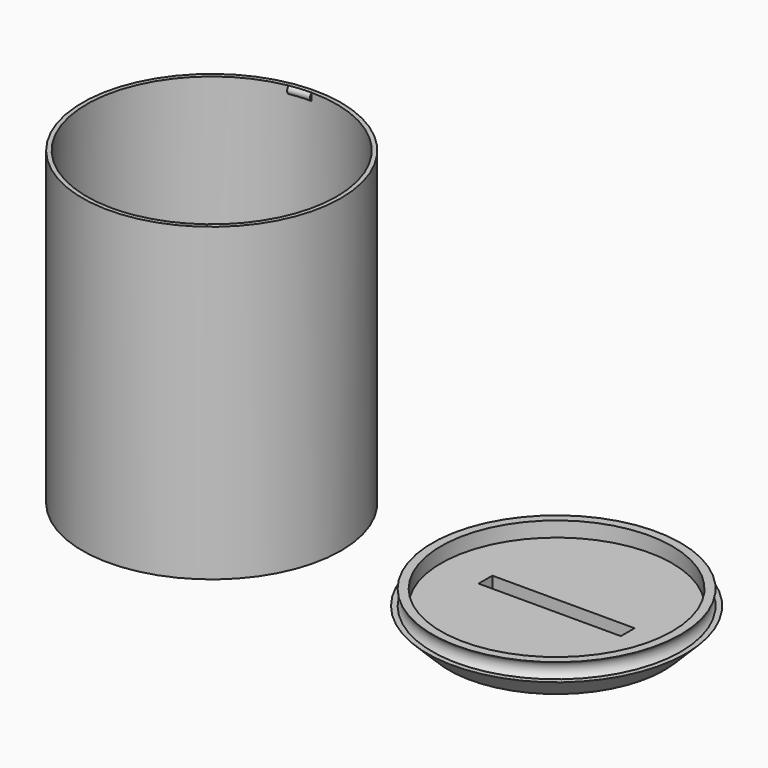
from build123d import *

# Parameters (mm, degrees)
F0_R          = 30
F1_DEPTH      = 2
F2_R          = 30
F2_R_2        = 29
F3_DEPTH      = 70
F5_ANGLE      = 10
F6_R          = 25
F7_DEPTH      = 5
F7_TAPER      = -45
F8_W          = 33
F8_H          = 4
F9_DEPTH      = 72.001
F10_R         = 28.8
F10_R_2       = 26.8
F11_DEPTH     = 3.5
F14_TEXT_SIZE = 3.9306186258
F15_DEPTH     = 1


# Not quite as in the source:
# - Text() gives the source's letters only with a copy of the font that has no kerning and outlines rounded to 1/6400 em; it was checked with that copy


with BuildPart() as f1:
    # F0 (on Top) → F1 (new body)
    with BuildSketch(Plane.XY):
        Circle(F0_R)
    extrude(amount=F1_DEPTH)

    # F2 (on face) → F3 (join)
    with BuildSketch(Plane.XY.offset(2)):
        Circle(F2_R)
        Circle(F2_R_2, mode=Mode.SUBTRACT)
    extrude(amount=F3_DEPTH)

    # F4 (on Right) → F5 (revolve)
    with BuildSketch(Plane.YZ):
        with BuildLine():
            Line((-29, 72), (-29, 70.2679491924))
            ThreePointArc((-29, 70.2679491924), (-28.5, 71.1339745962), (-29, 72))
        make_face()
        with BuildLine():
            Line((29, 70.2679491924), (29, 72))
            ThreePointArc((29, 72), (28.5, 71.1339745962), (29, 70.2679491924))
        make_face()
    revolve(axis=Axis((0, 0, 72), (0, 0, 1)), revolution_arc=F5_ANGLE)


with BuildPart() as f7:
    # F6 (on Top) → F7 (new body)
    with BuildSketch(Plane.XY):
        with Locations((80, 0)):
            Circle(F6_R)
    extrude(amount=F7_DEPTH, taper=F7_TAPER)

    # F8 (on face) → F9 (cut, through all)
    with BuildSketch(Plane(origin=(0, 0, 0), x_dir=(1, 0, 0), z_dir=(0, 0, -1))):
        with Locations((80, 0)):
            Rectangle(F8_W, F8_H)
    extrude(amount=-F9_DEPTH, mode=Mode.SUBTRACT)

    # F10 (on face) → F11 (join)
    with BuildSketch(Plane.XY.offset(5)):
        with Locations((80, 0)):
            Circle(F10_R)
        with Locations((80, 0)):
            Circle(F10_R_2, mode=Mode.SUBTRACT)
    extrude(amount=F11_DEPTH)

    # F12 (on Front) → F13 (revolve, cut)
    with BuildSketch(Plane.XZ):
        with BuildLine():
            ThreePointArc((108.8, 8.4871191548), (108, 6.7435595774), (108.8, 5))
            Line((108.8, 5), (108.8, 8.4871191548))
        make_face()
    revolve(axis=Axis((80, 0, 8.5), (0, 0, 1)), mode=Mode.SUBTRACT)

    # F14 (on face) → F15 (cut)
    with BuildSketch(Plane(origin=(0, 0, 0), x_dir=(1, 0, 0), z_dir=(0, 0, -1))):
        with Locations((63.5, 3)):
            Text('Saving money eh?', F14_TEXT_SIZE, font='Open Sans', text_align=(TextAlign.LEFT, TextAlign.BOTTOM))
        with Locations((64.6779572694, -5.8300454106)):
            Text("You've done well", F14_TEXT_SIZE, font='Open Sans', text_align=(TextAlign.LEFT, TextAlign.BOTTOM))
    extrude(amount=-F15_DEPTH, mode=Mode.SUBTRACT)


solid = Compound([f1.part, f7.part])
